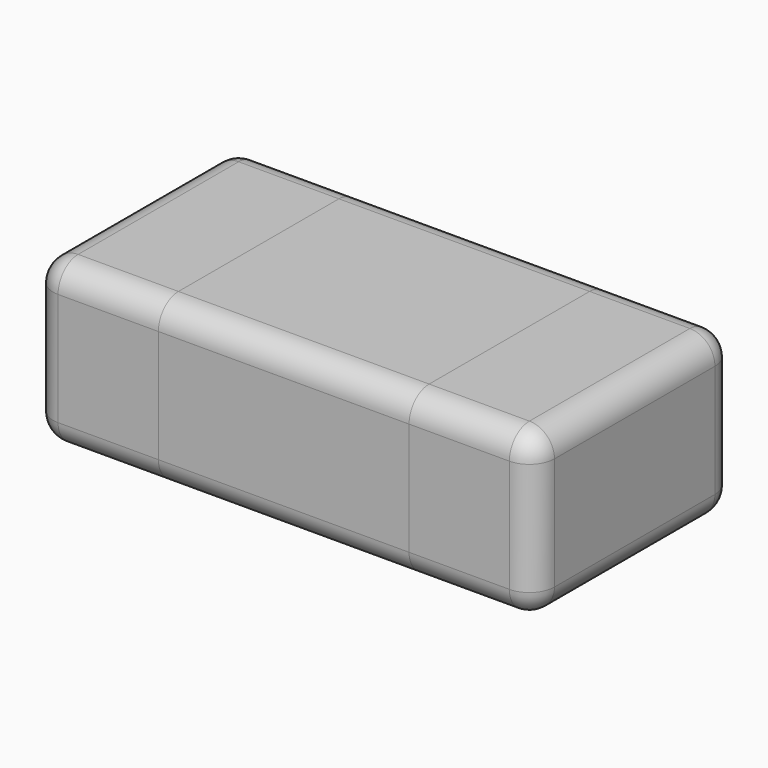
from build123d import *

# Parameters (mm, degrees)
F2_W     = 0.2
F2_H     = 0.2
F3_DEPTH = 0.11
F2_W_2   = 0.1
F4_DEPTH = 0.13
F5_DEPTH = 0.13
F6_DEPTH = 0.02
F7_R     = 0.01999
F7_2_R   = 0.01999
F7_3_R   = 0.01999
F7_4_R   = 0.01999


# Not quite as in the source:
# - a fillet or chamfer is up to 0.001 mm smaller than in the source, because OpenCascade refuses the exact size


with BuildPart() as f3:
    # F2 (on Top) → F3 (new body)
    with BuildSketch(Plane.XY):
        Rectangle(F2_W, F2_H)
    extrude(amount=F3_DEPTH)


with BuildPart() as f4:
    # F2 (on Top) → F4 (new body)
    with BuildSketch(Plane.XY):
        with Locations((-0.15, 0)):
            Rectangle(F2_W_2, F2_H)
    extrude(amount=F4_DEPTH)

    # F7 (radius 0.02 in the source; OpenCascade refuses exactly that, so slightly less here)
    f7_edges = [f4.edges().sort_by_distance(p)[0] for p in [
        (-0.15, -0.1, 0.13),
        (-0.2, 0.1, 0.065),
        (-0.2, -0.1, 0.065),
        (-0.2, 0, 0),
        (-0.2, 0, 0.13),
        (-0.15, 0.1, 0.13),
        (-0.15, 0.1, 0),
        (-0.15, -0.1, 0),
    ]]
    fillet(f7_edges, radius=F7_R)


with BuildPart() as f5:
    # F2 (on Top) → F5 (new body)
    with BuildSketch(Plane.XY):
        with Locations((0.15, 0)):
            Rectangle(F2_W_2, F2_H)
    extrude(amount=F5_DEPTH)

    # F7#2 (radius 0.02 in the source; OpenCascade refuses exactly that, so slightly less here)
    f7_2_edges = [f5.edges().sort_by_distance(p)[0] for p in [
        (0.15, -0.1, 0.13),
        (0.2, -0.1, 0.065),
        (0.2, 0.1, 0.065),
        (0.2, 0, 0),
        (0.2, 0, 0.13),
        (0.15, 0.1, 0.13),
        (0.15, 0.1, 0),
        (0.15, -0.1, 0),
    ]]
    fillet(f7_2_edges, radius=F7_2_R)


with BuildPart() as f6:
    # F6 (new): a face of the model
    f6_faces = [f3.part.faces().sort_by_distance(p)[0] for p in [
        (0, 0, 0.11),
    ]]
    extrude(f6_faces, amount=F6_DEPTH)

    # F7#4 (radius 0.02 in the source; OpenCascade refuses exactly that, so slightly less here)
    f7_4_edges = [f6.edges().sort_by_distance(p)[0] for p in [
        (0, -0.1, 0.13),
        (0, 0.1, 0.13),
    ]]
    fillet(f7_4_edges, radius=F7_4_R)


with BuildPart() as f3_1:
    add(f3.part)

    # F7#3 (radius 0.02 in the source; OpenCascade refuses exactly that, so slightly less here)
    f7_3_edges = [f3_1.edges().sort_by_distance(p)[0] for p in [
        (0, 0.1, 0),
        (0, -0.1, 0),
    ]]
    fillet(f7_3_edges, radius=F7_3_R)


solid = Compound([f4.part, f5.part, f6.part, f3_1.part])
